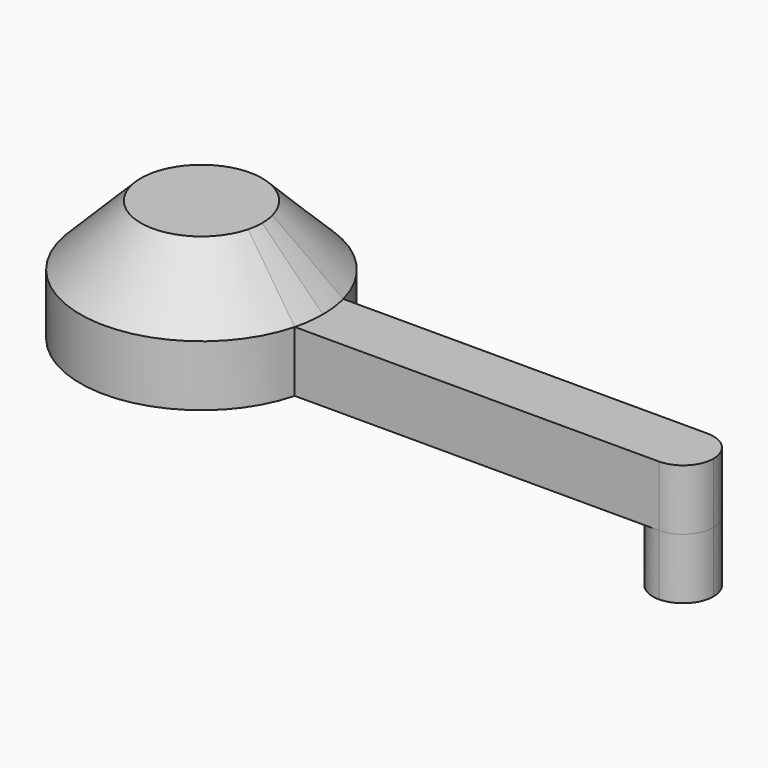
from build123d import *

# Parameters (mm, degrees)
F1_DEPTH = 6.35
F2_DEPTH = 3.175
F3_SIZE  = 3.17499
F4_DEPTH = 3.175


# Not quite as in the source:
# - a fillet or chamfer is up to 0.001 mm smaller than in the source, because OpenCascade refuses the exact size


with BuildPart() as f1:
    # F0 (on Top) → F1 (new body)
    with BuildSketch(Plane.XY):
        with BuildLine():
            Line((6.1483610621, 0), (6.1483610621, 1.5875))
            ThreePointArc((6.1483610621, 1.5875), (-6.35, 0), (6.1483610621, -1.5875))
            Line((6.1483610621, -1.5875), (6.1483610621, 0))
        make_face()
        with BuildLine():
            ThreePointArc((6.1483610621, -1.5875), (6.2993885713, -0.8001272573), (6.35, 0))
            ThreePointArc((6.35, 0), (6.2993885713, 0.8001272573), (6.1483610621, 1.5875))
            Line((6.1483610621, 1.5875), (6.1483610621, 0))
            Line((6.1483610621, 0), (6.1483610621, -1.5875))
        make_face()
    extrude(amount=F1_DEPTH)

    # F0 (on Top) → F2 (join)
    with BuildSketch(Plane.XY):
        with BuildLine():
            ThreePointArc((6.1483610621, 1.5875), (6.2993885713, 0.8001272573), (6.35, 0))
            ThreePointArc((6.35, 0), (6.2993885713, -0.8001272573), (6.1483610621, -1.5875))
            Line((6.1483610621, -1.5875), (25.1983610621, -1.5875))
            ThreePointArc((25.1983610621, -1.5875), (23.6108610621, 0), (25.1983610621, 1.5875))
            Line((25.1983610621, 1.5875), (6.1483610621, 1.5875))
        make_face()
        with BuildLine():
            ThreePointArc((26.7858610621, 0), (26.3208930772, 1.1225320151), (25.1983610621, 1.5875))
            Line((25.1983610621, 1.5875), (25.1983610621, -1.5875))
            ThreePointArc((25.1983610621, -1.5875), (26.3208930772, -1.1225320151), (26.7858610621, 0))
        make_face()
        with BuildLine():
            Line((25.1983610621, -1.5875), (25.1983610621, 1.5875))
            ThreePointArc((25.1983610621, 1.5875), (23.6108610621, 0), (25.1983610621, -1.5875))
        make_face()
    extrude(amount=F2_DEPTH)

    # F3 (size 3.175 in the source; OpenCascade refuses exactly that, so slightly less here)
    f3_edges = [f1.edges().sort_by_distance(p)[0] for p in [
        (-6.148361, 1.5875, 6.35),
    ]]
    chamfer(f3_edges, length=F3_SIZE)

    # F0 (on Top) → F4 (join)
    with BuildSketch(Plane.XY):
        with BuildLine():
            ThreePointArc((26.7858610621, 0), (26.3208930772, 1.1225320151), (25.1983610621, 1.5875))
            Line((25.1983610621, 1.5875), (25.1983610621, -1.5875))
            ThreePointArc((25.1983610621, -1.5875), (26.3208930772, -1.1225320151), (26.7858610621, 0))
        make_face()
        with BuildLine():
            Line((25.1983610621, -1.5875), (25.1983610621, 1.5875))
            ThreePointArc((25.1983610621, 1.5875), (23.6108610621, 0), (25.1983610621, -1.5875))
        make_face()
    extrude(amount=-F4_DEPTH)


solid = f1.part
